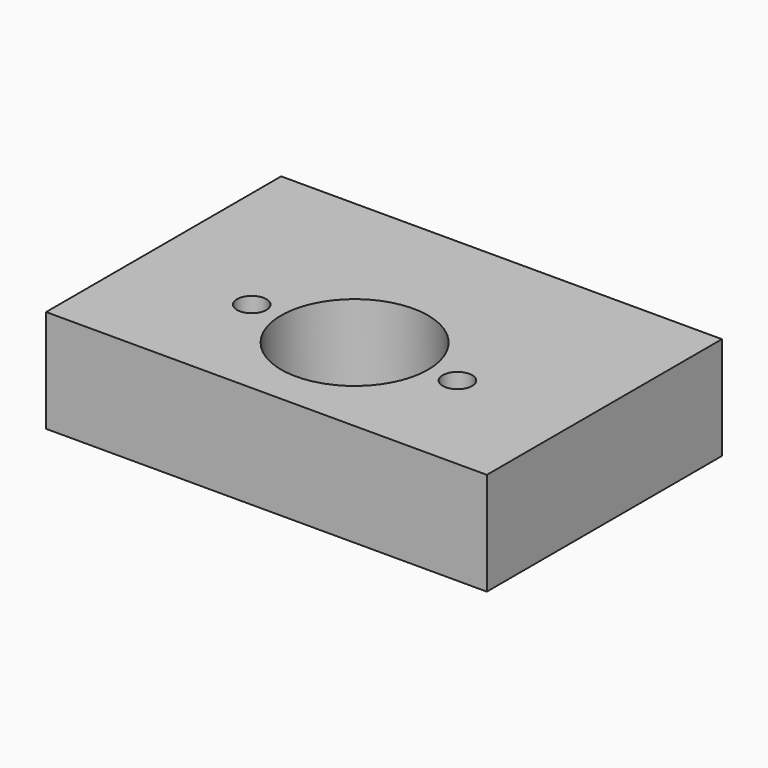
from build123d import *

# Parameters (mm, degrees)
F0_W     = 60
F0_H     = 40
F1_DEPTH = 14
F2_R     = 10
F2_R_2   = 2
F4_DEPTH = 14


# Not quite as in the source:
# - the program builds the solid bodies; features that only make, move or delete a surface that nothing else refers to are left out


with BuildPart() as f1:
    # F0 (on Top) → F1 (new body)
    with BuildSketch(Plane.XY):
        Rectangle(F0_W, F0_H)
    extrude(amount=-F1_DEPTH)

    # F2 (on face) → F4 (cut, through all)
    with BuildSketch(Plane.XY):
        with Locations((0, -5)):
            Circle(F2_R)
        with Locations((-14, -5)):
            Circle(F2_R_2)
        with Locations((14, -5)):
            Circle(F2_R_2)
    extrude(amount=-F4_DEPTH, mode=Mode.SUBTRACT)


solid = f1.part
